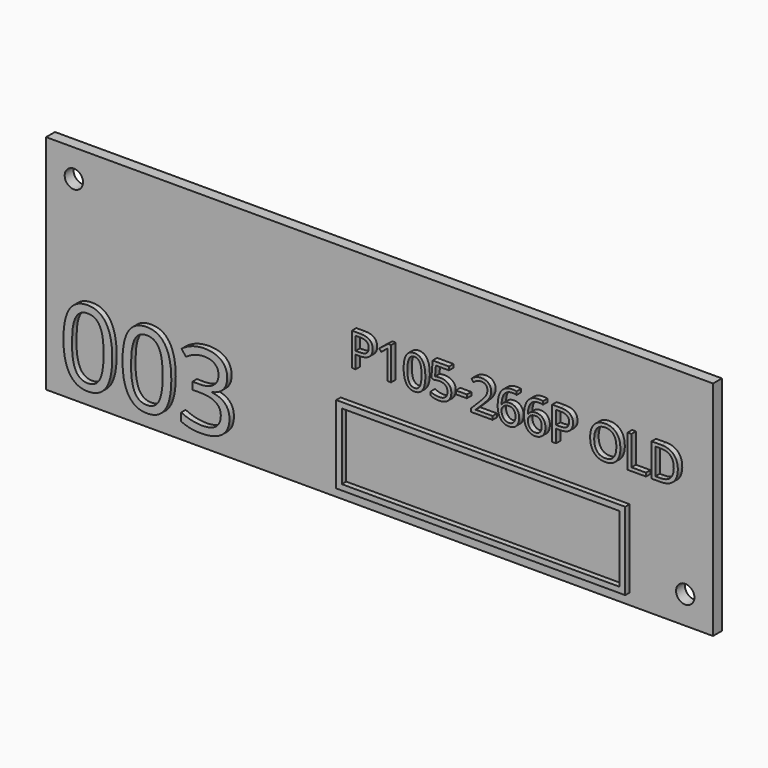
from build123d import *

# Parameters (mm, degrees)
F0_W         = 120
F0_H         = 40
F1_DEPTH     = 2
F3_D         = 3.3
F4_TEXT_SIZE = 8.2797878304
F5_DEPTH     = 1
F6_TEXT_SIZE = 18.5894526641
F7_DEPTH     = 1
F8_W         = 52
F8_H         = 14
F8_W_2       = 49.99999962
F8_H_2       = 11.99999962
F9_DEPTH     = 1


# Not quite as in the source:
# - Text() gives the source's letters only with a copy of the font that has no kerning and outlines rounded to 1/6400 em; it was checked with that copy


with BuildPart() as f1:
    # F0 (on Front) → F1 (new body)
    with BuildSketch(Plane.XZ):
        Rectangle(F0_W, F0_H)
    extrude(amount=F1_DEPTH)

    # F3 (through all)
    with Locations(Plane.XZ.offset(2)):
        with Locations((-55, 15), (55, -15)):
            Hole(F3_D / 2)

    # F4 (on face) → F5 (join)
    with BuildSketch(Plane.XZ.offset(2)):
        with Locations((-5, 2)):
            Text('P105-266P OLD', F4_TEXT_SIZE, font='Open Sans', text_align=(TextAlign.LEFT, TextAlign.BOTTOM))
    extrude(amount=F5_DEPTH)

    # F6 (on face) → F7 (join)
    with BuildSketch(Plane.XZ.offset(2)):
        with Locations((-57, -17)):
            Text('003', F6_TEXT_SIZE, font='Open Sans', text_align=(TextAlign.LEFT, TextAlign.BOTTOM))
    extrude(amount=F7_DEPTH)

    # F8 (on face) → F9 (join)
    with BuildSketch(Plane.XZ.offset(2)):
        with Locations((19, -11)):
            Rectangle(F8_W, F8_H)
        with Locations((19, -11)):
            Rectangle(F8_W_2, F8_H_2, mode=Mode.SUBTRACT)
    extrude(amount=F9_DEPTH)


solid = f1.part
